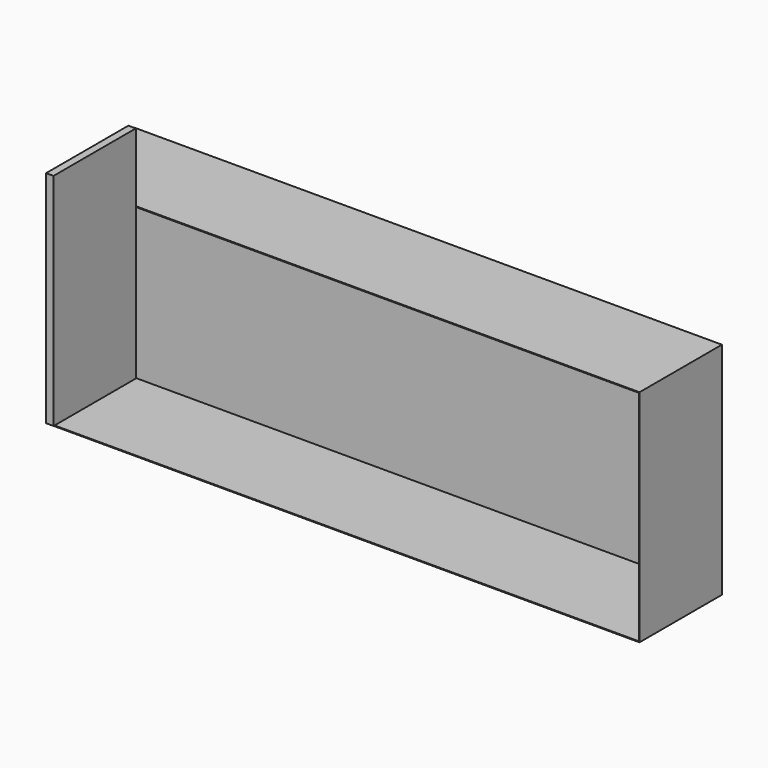
from build123d import *

# Parameters (mm, degrees)
F1_E0_TOP_W = 2000.00108
F1_E0_TOP_H = 350.52
F2_DEPTH    = 749.3
F3_T        = -2.54
F4_W        = 349.9993
F4_H        = 749.3
F5_DEPTH    = 25.4


with BuildPart() as f2:
    # F1_E0_top (on explicit) → F2 (new body)
    with BuildSketch(Plane(origin=(-995.5664890079, 0, -610.6151250599), x_dir=(1, 0, 0), z_dir=(0, 0, 1))):
        with Locations((1000.00054, 175.26)):
            Rectangle(F1_E0_TOP_W, F1_E0_TOP_H)
    extrude(amount=F2_DEPTH)

    # F3
    f3_openings = [f2.faces().sort_by_distance(p)[0] for p in [
        (4.434051, 0, -235.965125),
    ]]
    offset(amount=F3_T, openings=f3_openings)


with BuildPart() as f5:
    # F4 (on Right) → F5 (new body)
    with BuildSketch(Plane.YZ):
        with Locations((-1093.6340689659, 609.4311486613)):
            Rectangle(F4_W, F4_H)
    extrude(amount=F5_DEPTH)


solid = Compound([f2.part, f5.part])
